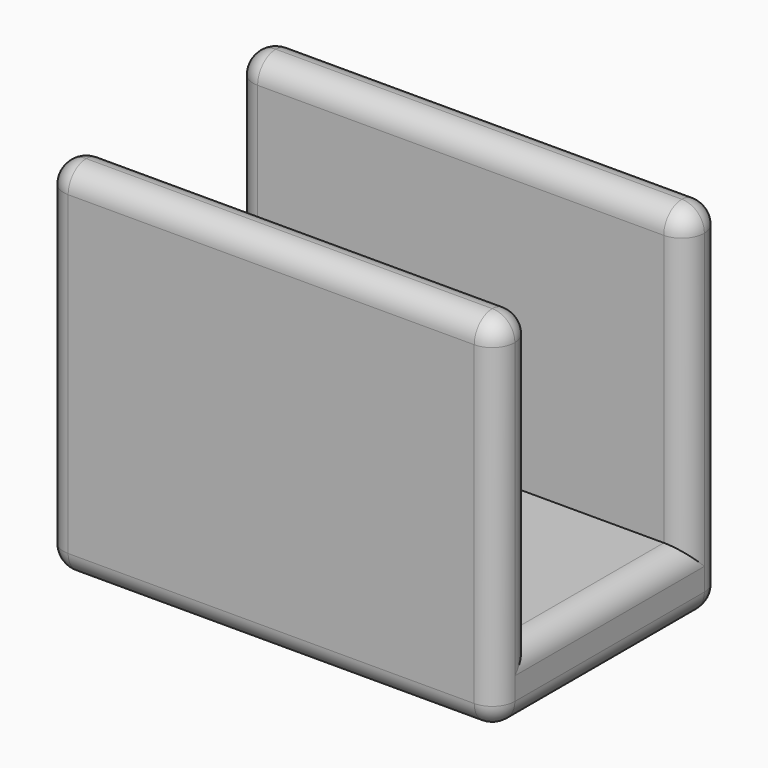
from build123d import *

# Parameters (mm, degrees)
F0_W     = 20
F0_H     = 2
F0_H_2   = 8.5
F1_DEPTH = 3
F2_DEPTH = 16
F3_R     = 0.99999


# Not quite as in the source:
# - a fillet or chamfer is up to 0.001 mm smaller than in the source, because OpenCascade refuses the exact size


with BuildPart() as f1:
    # F0 (on Top) → F1 (new body)
    with BuildSketch(Plane.XY):
        with Locations((10, -1)):
            Rectangle(F0_W, F0_H)
        with Locations((10, -6.25)):
            Rectangle(F0_W, F0_H_2)
        with Locations((10, -11.5)):
            Rectangle(F0_W, F0_H)
    extrude(amount=F1_DEPTH)

    # F0 (on Top) → F2 (join)
    with BuildSketch(Plane.XY):
        with Locations((10, -1)):
            Rectangle(F0_W, F0_H)
        with Locations((10, -11.5)):
            Rectangle(F0_W, F0_H)
    extrude(amount=F2_DEPTH)

    # F3 (radius 1 in the source; OpenCascade refuses exactly that, so slightly less here)
    f3_edges = [f1.edges().sort_by_distance(p)[0] for p in [
        (10, 0, 16),
        (0, -1, 16),
        (10, -2, 16),
        (20, -1, 16),
        (10, -10.5, 16),
        (0, -11.5, 16),
        (10, -12.5, 16),
        (20, -11.5, 16),
        (0, -6.25, 0),
        (0, 0, 8),
        (0, -2, 9.5),
        (0, -6.25, 3),
        (0, -10.5, 9.5),
        (0, -12.5, 8),
        (20, -6.25, 0),
        (20, -12.5, 8),
        (20, -10.5, 9.5),
        (20, -6.25, 3),
        (20, -2, 9.5),
        (20, 0, 8),
        (10, 0, 0),
        (10, -12.5, 0),
    ]]
    fillet(f3_edges, radius=F3_R)


solid = f1.part
